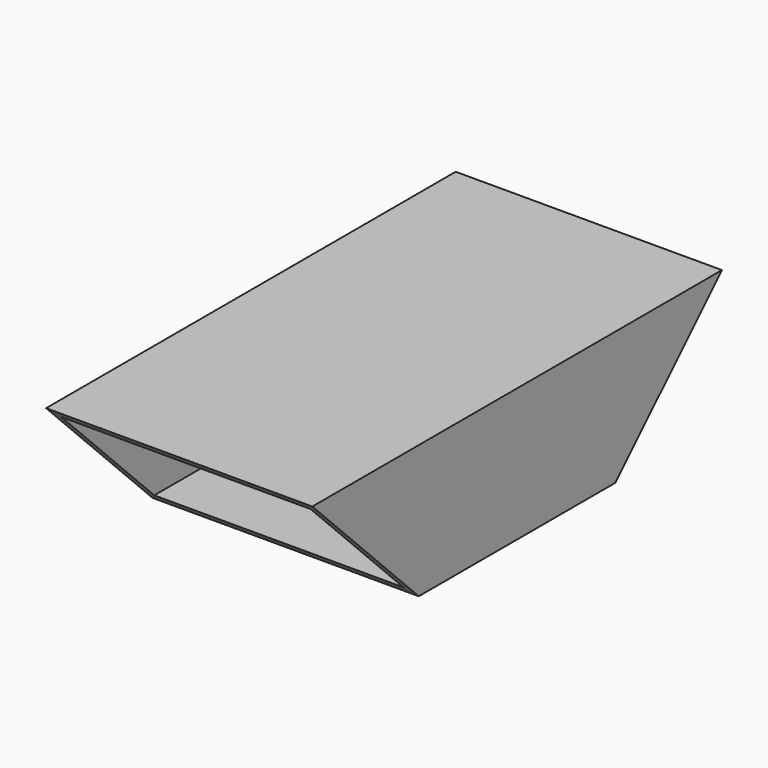
from build123d import *

# Parameters (mm, degrees)
F0_W        = 50
F0_H        = 25
F0_W_2      = 46.83
F0_H_2      = 21.83
F1_DEPTH    = 48.08
F2_T1_DEPTH = 178.5841493983
F3_T1_DEPTH = 178.5841493983


# Not quite as in the source:
# - a fillet or chamfer that OpenCascade refuses, or shapes differently, is made with other operations: its cross-section is extruded or revolved along the edge and cut away or added


with BuildPart() as f1:
    # F0 (on Front) → F1 (new body, symmetric)
    with BuildSketch(Plane.XZ):
        Rectangle(F0_W, F0_H)
        Rectangle(F0_W_2, F0_H_2, mode=Mode.SUBTRACT)
    extrude(amount=F1_DEPTH, both=True)

    # F2: chamfer of 25 on 1 edges, made by hand

    # F2_s2 → F2_t1 (cut)
    with BuildSketch(Plane.YZ.offset(-89.2920746991)):
        Polygon((-48.08, 12.5), (-23.08, -12.5), (-48.08, -12.5), align=None)
    extrude(amount=F2_T1_DEPTH, mode=Mode.SUBTRACT)

    # F3: chamfer of 25 on 1 edges, made by hand

    # F3_s2 → F3_t1 (cut)
    with BuildSketch(Plane.YZ.offset(-89.2920746991)):
        Polygon((23.08, -12.5), (48.08, 12.5), (48.08, -12.5), align=None)
    extrude(amount=F3_T1_DEPTH, mode=Mode.SUBTRACT)


solid = f1.part
